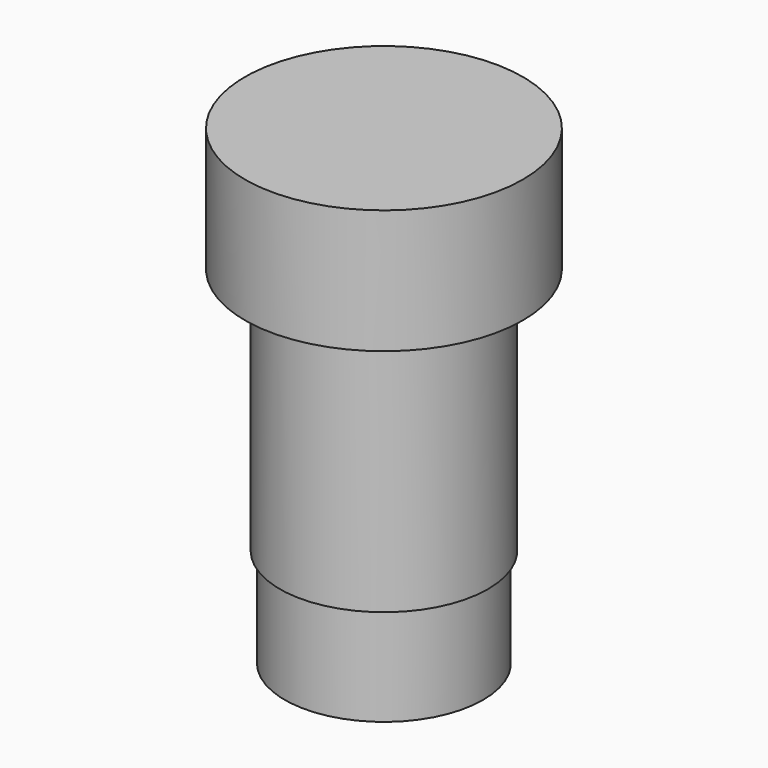
from build123d import *

# Parameters (mm, degrees)
F0_R     = 21
F0_R_2   = 20
F1_DEPTH = 50
F2_R     = 20
F3_DEPTH = 70
F2_R_2   = 28.0303533548
F2_R_3   = 21
F4_DEPTH = 25


with BuildPart() as f1:
    # F0 (on Top) → F1 (new body)
    with BuildSketch(Plane.XY):
        Circle(F0_R)
        Circle(F0_R_2, mode=Mode.SUBTRACT)
    extrude(amount=F1_DEPTH)


with BuildPart() as f3:
    # F2 (on face) → F3 (new body)
    with BuildSketch(Plane.XY.offset(50)):
        Circle(F2_R)
    extrude(amount=-F3_DEPTH)

    # F2 (on face) → F4 (join)
    with BuildSketch(Plane.XY.offset(50)):
        Circle(F2_R_2)
        Circle(F2_R_3, mode=Mode.SUBTRACT)
        Circle(F2_R_3)
        Circle(F2_R, mode=Mode.SUBTRACT)
        Circle(F2_R)
    extrude(amount=F4_DEPTH)


solid = Compound([f1.part, f3.part])
